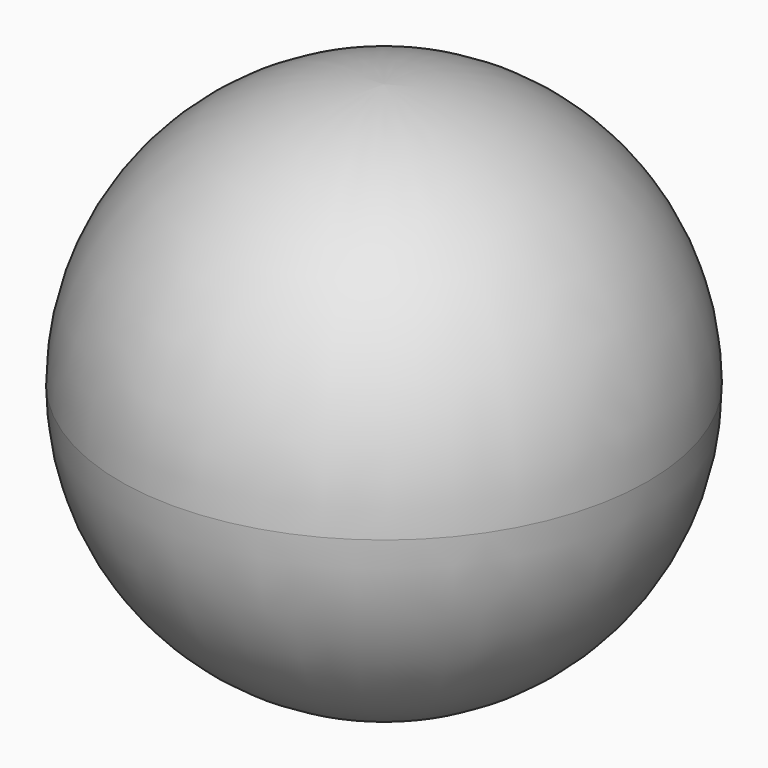
from build123d import *

# Parameters (mm, degrees)
F0_R     = 17.5
F1_DEPTH = 35
F2_R     = 17.49999


# Not quite as in the source:
# - a fillet or chamfer is up to 0.001 mm smaller than in the source, because OpenCascade refuses the exact size


with BuildPart() as f1:
    # F0 (on Top) → F1 (new body)
    with BuildSketch(Plane.XY):
        Circle(F0_R)
    extrude(amount=F1_DEPTH)

    # F2 (radius 17.5 in the source; OpenCascade refuses exactly that, so slightly less here)
    f2_edges = [f1.edges().sort_by_distance(p)[0] for p in [
        (-17.5, 0, 35),
        (-17.5, 0, 0),
    ]]
    fillet(f2_edges, radius=F2_R)


solid = f1.part
